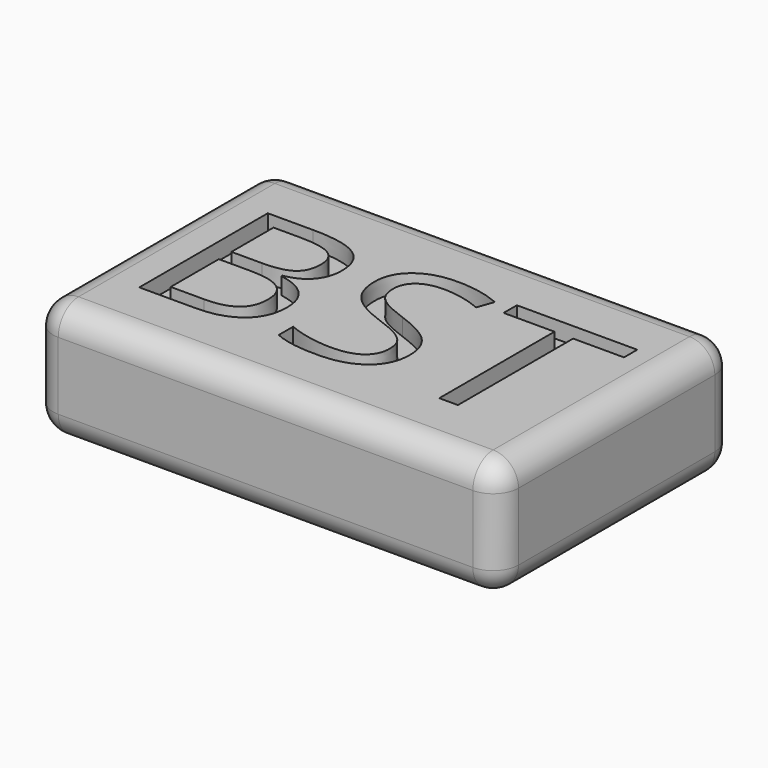
from build123d import *

# Parameters (mm, degrees)
F0_W         = 55
F0_H         = 35
F1_DEPTH     = 14
F2_R         = 3
F4_TEXT_SIZE = 26.5835929387
F5_DEPTH     = 2


# Not quite as in the source:
# - Text() gives the source's letters only with a copy of the font that has no kerning and outlines rounded to 1/6400 em; it was checked with that copy


with BuildPart() as f1:
    # F0 (on Top) → F1 (new body)
    with BuildSketch(Plane.XY):
        Rectangle(F0_W, F0_H)
    extrude(amount=F1_DEPTH)

    # F2
    f2_edges = [f1.edges().sort_by_distance(p)[0] for p in [
        (0, 17.5, 14),
        (0, -17.5, 14),
        (27.5, 0, 14),
        (-27.5, 0, 14),
        (0, -17.5, 0),
        (0, 17.5, 0),
        (-27.5, 0, 0),
        (27.5, 0, 0),
        (-27.5, -17.5, 7),
        (27.5, -17.5, 7),
        (27.5, 17.5, 7),
        (-27.5, 17.5, 7),
    ]]
    fillet(f2_edges, radius=F2_R)

    # F4 (on offset) → F5 (cut)
    with BuildSketch(Plane.XY.offset(14)):
        with Locations((-23.9068175313, -9.5271556544)):
            Text('BST', F4_TEXT_SIZE, font='Open Sans', text_align=(TextAlign.LEFT, TextAlign.BOTTOM))
    extrude(amount=-F5_DEPTH, mode=Mode.SUBTRACT)


solid = f1.part
